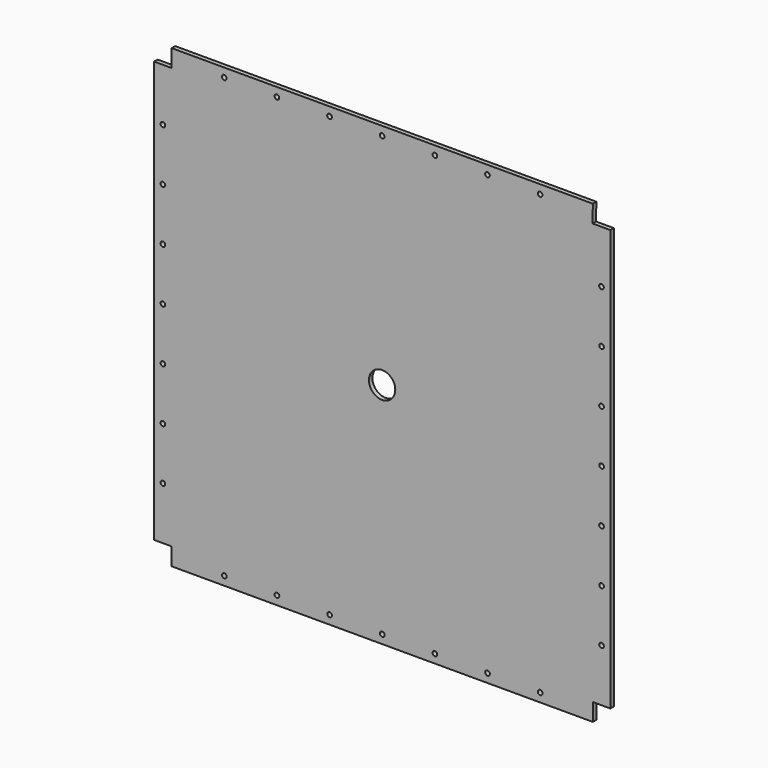
from build123d import *

# Parameters (mm, degrees)
F0_R     = 19.05
F1_DEPTH = 6.35
F2_D     = 6.7564
F2_DEPTH = 6.35
F2_TIP   = 2.0298273432


# Not quite as in the source:
# - ends of sketch curves that miss each other by under 0.0002 mm in the source are joined


with BuildPart() as f1:
    # F0 (on Front) → F1 (new body)
    with BuildSketch(Plane.XZ):
        Polygon((56.0273340809, 601.6124832813), (-553.5726659191, 601.6124832813), (-553.5710625288, 576.2108431508), (-578.9710624604, 576.2111164925), (-578.9710624604, -33.3878754139), (-553.5291783666, -33.3855858849), (-553.5726659191, -58.7875167187), (56.0273340809, -58.7875167187), (56.0289342467, -33.4404784252), (81.4289375396, -33.4404784254), (81.4289375396, 576.2111164925), (55.7141526242, 576.2144141151), align=None)
        with Locations((-248.9779856181, 271.4144141151)):
            Circle(F0_R, mode=Mode.SUBTRACT)
    extrude(amount=F1_DEPTH)

    # F2
    with Locations(Plane(origin=(0, 0, 0), x_dir=(1, 0, 0), z_dir=(0, 1, 0))):
        with Locations((-477.4505604353, -588.9118862284), (-401.2505604353, -588.8575930831), (-325.0505604353, -588.9123327142), (-248.8505604357, -588.9125559571), (-172.6505604357, -588.9127792), (-96.4505604357, -588.8575930831), (-20.2505604357, -588.9132256859), (68.5912178787, -500.010992039), (68.7289375396, -423.8111164925), (68.6305625245, -347.6111164925), (68.72896387, -271.4111800281), (68.6699071802, -195.2112029133), (68.7289375396, -119.0112029133), (68.7092518575, -42.8112054561), (-20.1613931545, 46.0873960761), (-96.3613931545, 46.0875217216), (-172.5613931536, 46.0871547073), (-248.7613931536, 46.0870340229), (-324.9613931536, 46.0869133385), (-401.1613931536, 46.0875167187), (-477.3613931536, 46.0866719696), (-566.2527381441, -42.8121245861), (-566.2710624604, -119.0121245861), (-566.2579736841, -195.2121245861), (-566.260591454, -271.4121245861), (-566.263209224, -347.6121245861), (-566.3166356603, -423.8121062841), (-566.2684447633, -500.0121062841)):
            Hole(F2_D / 2, depth=F2_DEPTH)
            with Locations((0, 0, -(F2_DEPTH + F2_TIP / 2))):  # 118° drill point
                Cone(0, F2_D / 2, F2_TIP, mode=Mode.SUBTRACT)


solid = f1.part
